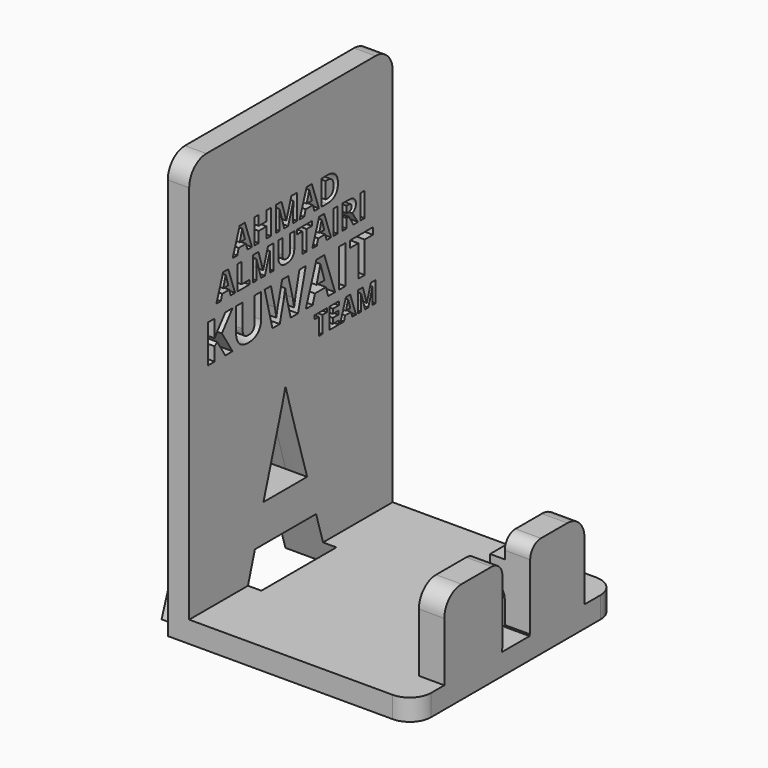
from build123d import *

# Parameters (mm, degrees)
F0_W          = 92
F0_H          = 95
F1_DEPTH      = 8
F2_W          = 8
F2_H          = 95
F3_DEPTH      = 150
F4_W          = 9.502086699
F4_H          = 65.4331929982
F5_DEPTH      = 30
F6_TEXT_SIZE  = 109.7222222222
F7_DEPTH      = 8
F8_DEPTH      = 13
F9_W          = 92.7244275808
F9_H          = 12.8235910088
F10_DEPTH     = 8
F11_T1_DEPTH  = 9.502086699
F11_T3_DEPTH  = 49.502086699
F11_T5_DEPTH  = 48
F11_T7_DEPTH  = 48
F11_T9_DEPTH  = 22.1511570575
F11_T11_DEPTH = 22.1686230261
F13_W         = 50
F13_H         = 8
F14_DEPTH     = 15
F15_W         = 13
F15_H         = 30
F16_DEPTH     = 51
F17_R         = 5
F21_TEXT_SIZE = 12.6808004755
F18_TEXT_SIZE = 19.8418849791
F19_TEXT_SIZE = 10.7493562003
F20_TEXT_SIZE = 13.037809648
F22_DEPTH     = 25
F23_R         = 5


# Not quite as in the source:
# - a fillet or chamfer that OpenCascade refuses, or shapes differently, is made with other operations: its cross-section is extruded or revolved along the edge and cut away or added
# - Text() gives the source's letters only with a copy of the font that has no kerning and outlines rounded to 1/6400 em; it was checked with that copy


with BuildPart() as f1:
    # F0 (on Top) → F1 (new body)
    with BuildSketch(Plane.XY):
        Rectangle(F0_W, F0_H)
    extrude(amount=F1_DEPTH)

    # F2 (on face) → F3 (join)
    with BuildSketch(Plane.XY.offset(8)):
        with Locations((-42, 0)):
            Rectangle(F2_W, F2_H)
    extrude(amount=F3_DEPTH)

    # F4 (on face) → F5 (join)
    with BuildSketch(Plane.XY.offset(8)):
        with Locations((41.2489566505, -0.6576199085)):
            Rectangle(F4_W, F4_H)
    extrude(amount=F5_DEPTH)

    # F6 (on face) → F7 (join)
    with BuildSketch(Plane(origin=(-46, 0, 0), x_dir=(0, -1, 0), z_dir=(-1, 0, 0))):
        with Locations((-35.3231336806, 0)):
            Text('A', F6_TEXT_SIZE, font='Open Sans', font_style=FontStyle.BOLD, text_align=(TextAlign.LEFT, TextAlign.BOTTOM))
    extrude(amount=F7_DEPTH)

    # F8 (cut): faces of the model
    f8_faces = [f1.faces().sort_by_distance(p)[0] for p in [
        (-46, -2.6092958686, 43.7110655024),
        (-46, -2.5310329861, 8.8111101838),
    ]]
    extrude(f8_faces, amount=-F8_DEPTH, mode=Mode.SUBTRACT)

    # F9 (on face) → F10 (cut)
    with BuildSketch(Plane.XY.offset(8)):
        Rectangle(F9_W, F9_H)
    extrude(amount=F10_DEPTH, mode=Mode.SUBTRACT)

    # F11: fillet of radius 8 on 10 edges, made by hand

    # F11_s2 → F11_t1 (join)
    with BuildSketch(Plane.YZ.offset(36.497913301)):
        with BuildLine():
            ThreePointArc((1.5882044956, 16), (-4.0686497539, 13.6568542495), (-6.4117955044, 8))
            Line((-6.4117955044, 8), (-6.4117955044, 16))
            Line((-6.4117955044, 16), (1.5882044956, 16))
        make_face()
        with BuildLine():
            ThreePointArc((6.4117955044, 8), (4.0686497539, 13.6568542495), (-1.5882044956, 16))
            Line((-1.5882044956, 16), (6.4117955044, 16))
            Line((6.4117955044, 16), (6.4117955044, 8))
        make_face()
    extrude(amount=F11_T1_DEPTH)

    # F11_s4 → F11_t3 (cut)
    with BuildSketch(Plane.YZ.offset(16.497913301)):
        with BuildLine():
            ThreePointArc((-33.3742164075, 30), (-31.031070657, 35.6568542495), (-25.3742164075, 38))
            Line((-25.3742164075, 38), (-33.3742164075, 38))
            Line((-33.3742164075, 38), (-33.3742164075, 30))
        make_face()
        with BuildLine():
            ThreePointArc((24.0589765906, 38), (29.7158308401, 35.6568542495), (32.0589765906, 30))
            Line((32.0589765906, 30), (32.0589765906, 38))
            Line((32.0589765906, 38), (24.0589765906, 38))
        make_face()
    extrude(amount=F11_T3_DEPTH, mode=Mode.SUBTRACT)

    # F11_s6 → F11_t5 (cut)
    with BuildSketch(Plane.XY.offset(-20)):
        with BuildLine():
            ThreePointArc((38, -47.5), (43.6568542495, -45.1568542495), (46, -39.5))
            Line((46, -39.5), (46, -47.5))
            Line((46, -47.5), (38, -47.5))
        make_face()
        with BuildLine():
            ThreePointArc((38, 47.5), (43.6568542495, 45.1568542495), (46, 39.5))
            Line((46, 39.5), (46, 47.5))
            Line((46, 47.5), (38, 47.5))
        make_face()
    extrude(amount=F11_T5_DEPTH, mode=Mode.SUBTRACT)

    # F11_s8 → F11_t7 (cut)
    with BuildSketch(Plane.YZ.offset(-66)):
        with BuildLine():
            ThreePointArc((47.5, 150), (45.1568542495, 155.6568542495), (39.5, 158))
            Line((39.5, 158), (47.5, 158))
            Line((47.5, 158), (47.5, 150))
        make_face()
        with BuildLine():
            ThreePointArc((-47.5, 150), (-45.1568542495, 155.6568542495), (-39.5, 158))
            Line((-39.5, 158), (-47.5, 158))
            Line((-47.5, 158), (-47.5, 150))
        make_face()
    extrude(amount=F11_T7_DEPTH, mode=Mode.SUBTRACT)

    # F11_s10 → F11_t9 (cut)
    with BuildSketch(Plane.YZ.offset(-68.1511570575)):
        with BuildLine():
            ThreePointArc((-6.968443427, 78.6571180556), (-11.5892092127, 77.1877017625), (-14.5125178655, 73.3192489439))
            Line((-14.5125178655, 73.3192489439), (-12.62890625, 78.6571180556))
            Line((-12.62890625, 78.6571180556), (-6.968443427, 78.6571180556))
        make_face()
    extrude(amount=F11_T9_DEPTH, mode=Mode.SUBTRACT)

    # F11_s12 → F11_t11 (cut)
    with BuildSketch(Plane.YZ.offset(-68.1686230261)):
        with BuildLine():
            ThreePointArc((9.5494221686, 73.3104701901), (6.6268195719, 77.1850127038), (2.0022556507, 78.6571180556))
            Line((2.0022556507, 78.6571180556), (7.6697048611, 78.6571180556))
            Line((7.6697048611, 78.6571180556), (9.5494221686, 73.3104701901))
        make_face()
    extrude(amount=F11_T11_DEPTH, mode=Mode.SUBTRACT)

    # F13 (on face) → F14 (join)
    with BuildSketch(Plane.YZ.offset(46)):
        with Locations((-0.3742164075, 26)):
            Rectangle(F13_W, F13_H)
    extrude(amount=-F14_DEPTH)

    # F15 (on Right) → F16 (cut)
    with BuildSketch(Plane.YZ):
        with Locations((0.2138538808, 23.445661515)):
            Rectangle(F15_W, F15_H)
    extrude(amount=F16_DEPTH, mode=Mode.SUBTRACT)

    # F17
    f17_edges = [f1.edges().sort_by_distance(p)[0] for p in [
        (41.248957, -6.286146, 38),
        (41.248957, 6.713854, 38),
    ]]
    fillet(f17_edges, radius=F17_R)

    # F21 (on face) + F18 (on face) + F19 (on face) + F20 (on face) → F22 (cut)
    with BuildSketch(Plane.YZ.offset(-38)):
        with Locations((-34.8122259855, 106.7333307635)):
            Text('ALMUTAIRI', F21_TEXT_SIZE, font='Open Sans', font_style=FontStyle.BOLD, text_align=(TextAlign.LEFT, TextAlign.BOTTOM))
    with BuildSketch(Plane.YZ.offset(-38)):
        with Locations((-40.433262405, 88.0184907196)):
            Text('KUWAIT', F18_TEXT_SIZE, font='Open Sans', font_style=FontStyle.BOLD, text_align=(TextAlign.LEFT, TextAlign.BOTTOM))
    with BuildSketch(Plane.YZ.offset(-38)):
        with Locations((10.734507814, 76.6298472881)):
            Text('TEAM', F19_TEXT_SIZE, font='Open Sans', font_style=FontStyle.BOLD, text_align=(TextAlign.LEFT, TextAlign.BOTTOM))
    with BuildSketch(Plane.YZ.offset(-38)):
        with Locations((-27.1967503495, 118.6231198336)):
            Text('AHMAD', F20_TEXT_SIZE, font='Open Sans', font_style=FontStyle.BOLD, text_align=(TextAlign.LEFT, TextAlign.BOTTOM))
    extrude(amount=-F22_DEPTH, mode=Mode.SUBTRACT)

    # F23
    f23_edges = [f1.edges().sort_by_distance(p)[0] for p in [
        (36.497913, 15.669819, 22),
        (36.497913, -15.830181, 22),
    ]]
    fillet(f23_edges, radius=F23_R)


solid = f1.part
